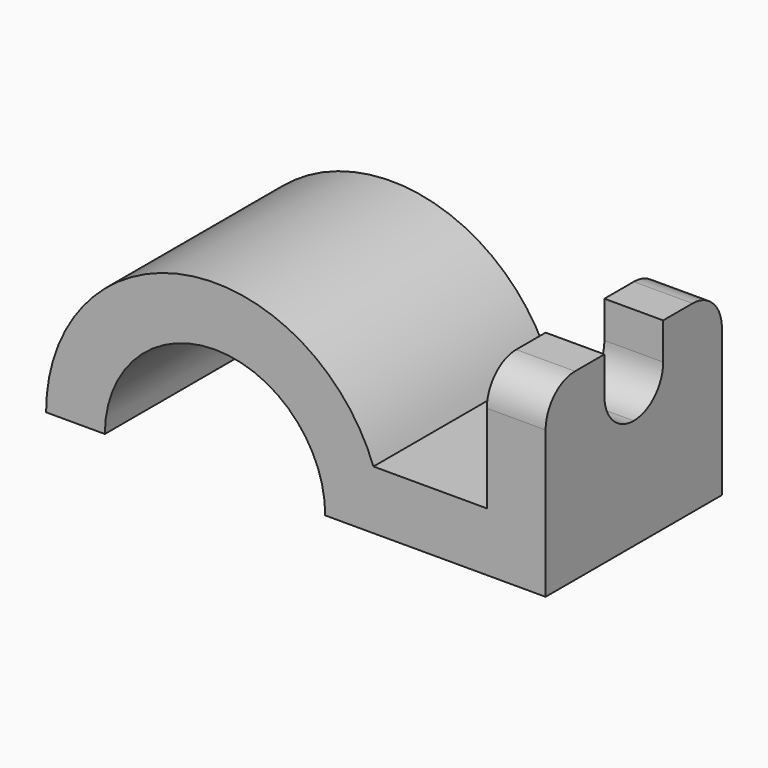
from build123d import *

# Parameters (mm, degrees)
F1_DEPTH = 30
F2_W     = 10
F2_H     = 10
F3_DEPTH = 8
F4_R     = 4.99999


# Not quite as in the source:
# - a fillet or chamfer is up to 0.001 mm smaller than in the source, because OpenCascade refuses the exact size


with BuildPart() as f1:
    # F0 (on Front) → F1 (new body)
    with BuildSketch(Plane.XZ):
        with BuildLine():
            ThreePointArc((-15, 0), (0, 15), (15, 0))
            Line((15, 0), (45, 0))
            Line((45, 0), (45, 25))
            Line((45, 25), (37, 25))
            Line((37, 25), (37, 8))
            Line((37, 8), (21.5638586528, 8))
            ThreePointArc((21.5638586528, 8), (-4.0639421123, 22.6381177333), (-23, 0))
            Line((-23, 0), (-15, 0))
        make_face()
    extrude(amount=F1_DEPTH)

    # F2 (on face) → F3 (cut, through all)
    with BuildSketch(Plane.YZ.offset(45)):
        with Locations((-15, 20)):
            Rectangle(F2_W, F2_H)
    extrude(amount=-F3_DEPTH, mode=Mode.SUBTRACT)

    # F4 (radius 5 in the source; OpenCascade refuses exactly that, so slightly less here)
    f4_edges = [f1.edges().sort_by_distance(p)[0] for p in [
        (41, -30, 25),
        (41, 0, 25),
        (41, -10, 15),
        (41, -20, 15),
    ]]
    fillet(f4_edges, radius=F4_R)


solid = f1.part
